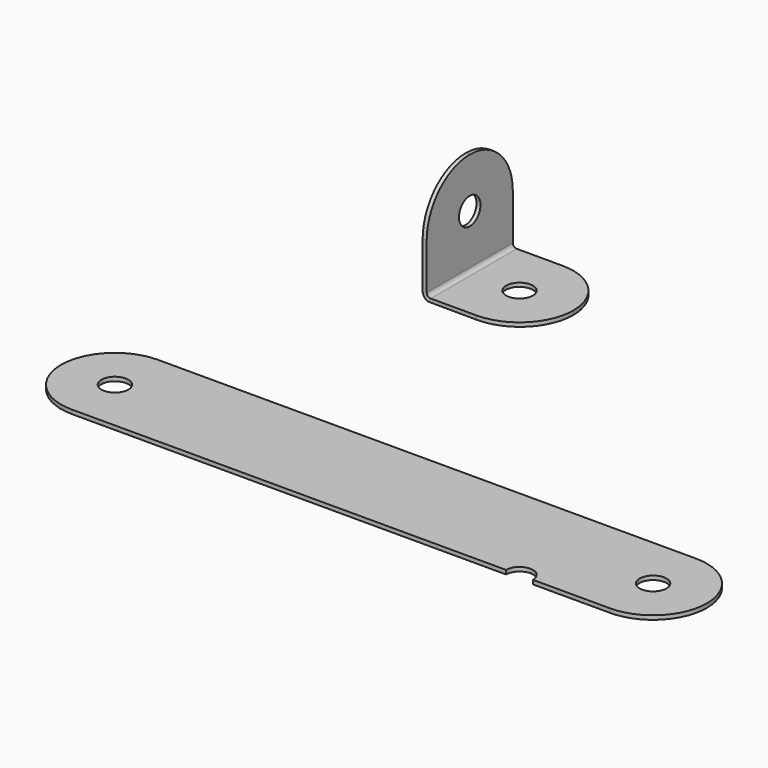
from build123d import *

# Parameters (mm, degrees)
F0_R     = 2.5
F1_DEPTH = 0.75
F3_DEPTH = 20
F5_D     = 5
F5_2_D   = 5
F7_D     = 5
F8_R     = 9.99999


# Not quite as in the source:
# - a fillet or chamfer is up to 0.001 mm smaller than in the source, because OpenCascade refuses the exact size


with BuildPart() as f1:
    # F0 (on Top) → F1 (new body)
    with BuildSketch(Plane.XY):
        with BuildLine():
            ThreePointArc((50, -10), (60, 0), (50, 10))
            Line((50, 10), (-50, 10))
            ThreePointArc((-50, 10), (-60, 0), (-50, -10))
            Line((-50, -10), (50, -10))
        make_face()
        with Locations((-50, 0)):
            Circle(F0_R, mode=Mode.SUBTRACT)
        with Locations((50, 0)):
            Circle(F0_R, mode=Mode.SUBTRACT)
    extrude(amount=F1_DEPTH)

    # F5 (through all)
    with Locations(Plane.XY.offset(47.2566441149)):
        with Locations((33.1826669741, -10)):
            Hole(F5_D / 2)


with BuildPart() as f3:
    # F2 (on Front) → F3 (new body)
    with BuildSketch(Plane.XZ):
        with BuildLine():
            Line((43.1826669741, 47.2566441149), (24.6826669741, 47.2566441149))
            ThreePointArc((24.6826669741, 47.2566441149), (24.1523368882, 47.476314029), (23.9326669741, 48.0066441149))
            Line((23.9326669741, 48.0066441149), (23.9326669741, 66.5066441149))
            Line((23.9326669741, 66.5066441149), (23.1826669741, 66.5066441149))
            Line((23.1826669741, 66.5066441149), (23.1826669741, 48.0066441149))
            ThreePointArc((23.1826669741, 48.0066441149), (23.4559897983, 47.1433578897), (24.176351116, 46.5946794369))
            Line((24.176351116, 46.5946794369), (43.1826669741, 46.5066441149))
            Line((43.1826669741, 46.5066441149), (43.1826669741, 47.2566441149))
        make_face()
    extrude(amount=F3_DEPTH)

    # F5#2 (through all)
    with Locations(Plane.XY.offset(47.2566441149)):
        with Locations((33.1826669741, -10)):
            Hole(F5_2_D / 2)

    # F7 (through all)
    with Locations(Plane.YZ.offset(23.9326669741)):
        with Locations((-10, 57.2566441149)):
            Hole(F7_D / 2)

    # F8 (radius 10 in the source; OpenCascade refuses exactly that, so slightly less here)
    f8_edges = [f3.edges().sort_by_distance(p)[0] for p in [
        (23.557667, -20, 66.506644),
        (23.557667, 0, 66.506644),
        (43.182667, -20, 46.881644),
        (43.182667, 0, 46.881644),
    ]]
    fillet(f8_edges, radius=F8_R)


solid = Compound([f1.part, f3.part])
